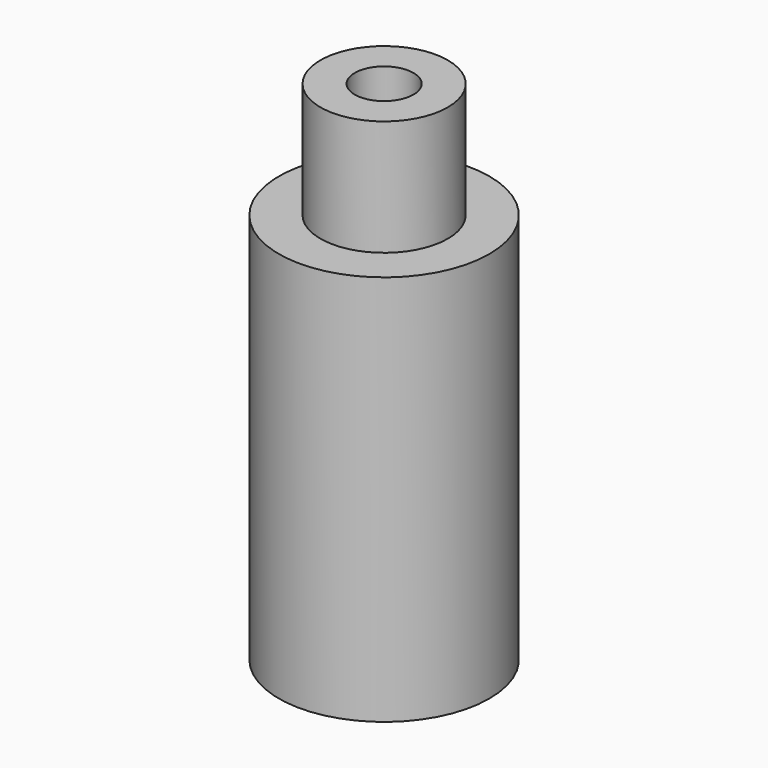
from build123d import *

# Parameters (mm, degrees)
F0_R     = 3.7338
F1_DEPTH = 13.8811
F2_R     = 2.2606
F3_DEPTH = 4.1021
F4_R     = 1.0414
F5_DEPTH = 47.0154
F6_R     = 2.53873
F7_DEPTH = 12.6492
F8_R     = 3.7338
F9_DEPTH = 13.5382


with BuildPart() as f1:
    # F0 (on Top) → F1 (new body)
    with BuildSketch(Plane.XY):
        Circle(F0_R)
    extrude(amount=F1_DEPTH)

    # F2 (on face) → F3 (join)
    with BuildSketch(Plane.XY.offset(13.8811)):
        Circle(F2_R)
    extrude(amount=F3_DEPTH)

    # F4 (on face) → F5 (cut)
    with BuildSketch(Plane.XY.offset(17.9832)):
        Circle(F4_R)
    extrude(amount=-F5_DEPTH, mode=Mode.SUBTRACT)

    # F6 (on face) → F7 (cut)
    with BuildSketch(Plane(origin=(0, 0, 0), x_dir=(1, 0, 0), z_dir=(0, 0, -1))):
        Circle(F6_R)
    extrude(amount=-F7_DEPTH, mode=Mode.SUBTRACT)

    # F8 (on face) → F9 (join)
    with BuildSketch(Plane(origin=(0, 0, 0), x_dir=(1, 0, 0), z_dir=(0, 0, -1))):
        Circle(F8_R)
        with BuildLine():
            Line((1.1798710111, 2.2479), (2.2479, 2.2479))
            Line((2.2479, 2.2479), (2.2479, 1.1798710111))
            ThreePointArc((2.2479, 1.1798710111), (2.4649504234, 0.6075931393), (2.53873, 0))
            ThreePointArc((2.53873, 0), (2.4649504234, -0.6075931393), (2.2479, -1.1798710111))
            Line((2.2479, -1.1798710111), (2.2479, -2.2479))
            Line((2.2479, -2.2479), (1.1798710111, -2.2479))
            ThreePointArc((1.1798710111, -2.2479), (0, -2.53873), (-1.1798710111, -2.2479))
            Line((-1.1798710111, -2.2479), (-2.2479, -2.2479))
            Line((-2.2479, -2.2479), (-2.2479, -1.1798710111))
            ThreePointArc((-2.2479, -1.1798710111), (-2.53873, 0), (-2.2479, 1.1798710111))
            Line((-2.2479, 1.1798710111), (-2.2479, 2.2479))
            Line((-2.2479, 2.2479), (-1.1798710111, 2.2479))
            ThreePointArc((-1.1798710111, 2.2479), (0, 2.53873), (1.1798710111, 2.2479))
        make_face(mode=Mode.SUBTRACT)
        with BuildLine():
            Line((-1.1798710111, 2.2479), (1.1798710111, 2.2479))
            ThreePointArc((1.1798710111, 2.2479), (0, 2.53873), (-1.1798710111, 2.2479))
        make_face()
        with BuildLine():
            ThreePointArc((2.53873, 0), (2.4649504234, 0.6075931393), (2.2479, 1.1798710111))
            Line((2.2479, 1.1798710111), (2.2479, -1.1798710111))
            ThreePointArc((2.2479, -1.1798710111), (2.4649504234, -0.6075931393), (2.53873, 0))
        make_face()
        with BuildLine():
            Line((-2.2479, -1.1798710111), (-2.2479, 1.1798710111))
            ThreePointArc((-2.2479, 1.1798710111), (-2.53873, 0), (-2.2479, -1.1798710111))
        make_face()
        with BuildLine():
            ThreePointArc((-1.1798710111, -2.2479), (0, -2.53873), (1.1798710111, -2.2479))
            Line((1.1798710111, -2.2479), (-1.1798710111, -2.2479))
        make_face()
    extrude(amount=-F9_DEPTH)


solid = f1.part
